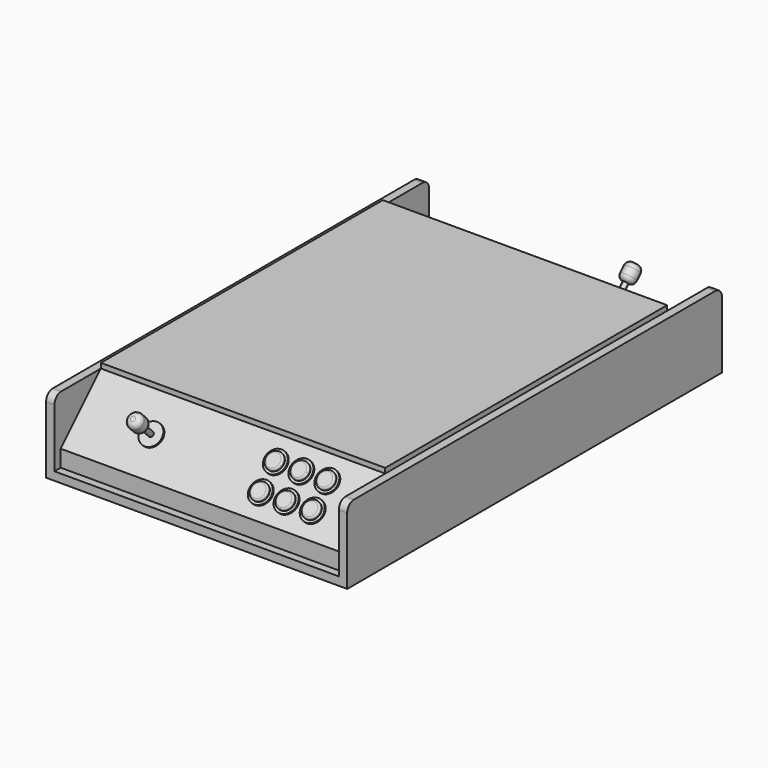
from build123d import *

# Parameters (mm, degrees)
F0_W      = 457.2
F0_H      = 711.2
F1_DEPTH  = 12.7
F3_DEPTH  = 101.6
F4_W      = 431.8
F4_H      = 171.8578838676
F5_DEPTH  = 101.6
F6_SIZE   = 76.2
F7_R      = 12.7
F8_SIZE   = 76.2
F9_R      = 12.7
F11_R     = 16.51
F11_R_2   = 12.7
F12_DEPTH = 2.54
F13_DEPTH = 7.62
F14_R     = 2.54
F15_DEPTH = 2.54
F16_DEPTH = 25.4
F17_R     = 11.120165797
F18_DEPTH = 25.4
F20_R     = 16.51
F20_R_2   = 12.7
F21_DEPTH = 2.54
F22_DEPTH = 7.62
F23_R     = 2.54
F24_DEPTH = 2.54
F25_DEPTH = 25.4
F26_R     = 11.1201708
F27_DEPTH = 25.4
F10_W     = 431.8
F10_H     = 496.0420746356
F29_DEPTH = 101.6
F30_W     = 412.6160778105
F30_H     = 477.2938070819
F31_DEPTH = 101.6
F32_SIZE2 = 61.2531853898
F32_SIZE  = 228.6
F33_W     = 431.8
F33_H     = 535.0315354705
F34_DEPTH = 7.62


# Not quite as in the source:
# - a fillet or chamfer that OpenCascade refuses, or shapes differently, is made with other operations: its cross-section is extruded or revolved along the edge and cut away or added


with BuildPart() as f1:
    # F0 (on Top) → F1 (new body)
    with BuildSketch(Plane.XY):
        with Locations((-174.0402644813, 227.3841096222)):
            Rectangle(F0_W, F0_H)
    extrude(amount=F1_DEPTH)

    # F2 (on face) → F3 (join)
    with BuildSketch(Plane.XY.offset(12.7)):
        Polygon((54.5597355187, 570.2841096222), (54.5597355187, 582.9841096222), (41.8597355187, 582.9841096222), (41.8597355187, -128.2158903778), (54.5597355187, -128.2158903778), (54.5597355187, -115.5158903778), align=None)
        Polygon((-389.9402644813, 582.9841096222), (-402.6402644813, 582.9841096222), (-402.6402644813, 570.2841096222), (-402.6402644813, -115.5158903778), (-402.6402644813, -128.2158903778), (-389.9402644813, -128.2158903778), align=None)
    extrude(amount=F3_DEPTH)

    # F4 (on face) → F5 (join)
    with BuildSketch(Plane.XY.offset(12.7)):
        with Locations((-174.0402644813, 485.1709354237)):
            Rectangle(F4_W, F4_H)
        Polygon((41.8597355187, 227.3841096222), (41.8597355187, 399.2419934899), (-389.9402644813, 399.2419934899), (-389.9402644813, 227.3841096222), (-389.9402644813, 55.5262257546), (41.8597355187, 55.5262257546), align=None)
        with Locations((-174.0402644813, -30.4027161792)):
            Rectangle(F4_W, F4_H)
    extrude(amount=F5_DEPTH)

    # F6
    f6_edges = [f1.edges().sort_by_distance(p)[0] for p in [
        (-174.040264, 571.099877, 114.3),
    ]]
    chamfer(f6_edges, length=F6_SIZE)

    # F7
    f7_edges = [f1.edges().sort_by_distance(p)[0] for p in [
        (-396.290264, 582.98411, 114.3),
        (48.209736, 582.98411, 114.3),
    ]]
    fillet(f7_edges, radius=F7_R)

    # F8
    f8_edges = [f1.edges().sort_by_distance(p)[0] for p in [
        (-174.040264, -116.331658, 114.3),
    ]]
    chamfer(f8_edges, length=F8_SIZE)

    # F9
    f9_edges = [f1.edges().sort_by_distance(p)[0] for p in [
        (-396.290264, -128.21589, 114.3),
        (48.209736, -128.21589, 114.3),
    ]]
    fillet(f9_edges, radius=F9_R)

    # F11 (on face) → F12 (join)
    with BuildSketch(Plane(origin=(0, 304.5999386787, 304.5999386787), x_dir=(-1, 0, 0), z_dir=(0, 0.7071067812, 0.7071067812))):
        with Locations((245.9873259068, -301.1169731617)):
            Circle(F11_R)
        with Locations((245.9873259068, -301.1169731617)):
            Circle(F11_R_2, mode=Mode.SUBTRACT)
        with BuildLine():
            ThreePointArc((298.5002644813, -301.1169731617), (293.6645974387, -289.4426402043), (281.9902644813, -284.6069731617))
            Line((281.9902644813, -284.6069731617), (281.9902644813, -288.4169731617))
            ThreePointArc((281.9902644813, -288.4169731617), (290.9705206024, -292.1367170406), (294.6902644813, -301.1169731617))
            ThreePointArc((294.6902644813, -301.1169731617), (290.9705206024, -310.0972292828), (281.9902644813, -313.8169731617))
            Line((281.9902644813, -313.8169731617), (281.9902644813, -317.6269731617))
            ThreePointArc((281.9902644813, -317.6269731617), (293.6645974387, -312.7913061191), (298.5002644813, -301.1169731617))
        make_face()
        with BuildLine():
            Line((281.9902644813, -288.4169731617), (281.9902644813, -284.6069731617))
            ThreePointArc((281.9902644813, -284.6069731617), (265.4802644813, -301.1169731617), (281.9902644813, -317.6269731617))
            Line((281.9902644813, -317.6269731617), (281.9902644813, -313.8169731617))
            ThreePointArc((281.9902644813, -313.8169731617), (269.2902644813, -301.1169731617), (281.9902644813, -288.4169731617))
        make_face()
        with Locations((319.3984925747, -301.1169731617)):
            Circle(F11_R)
        with Locations((319.3984925747, -301.1169731617)):
            Circle(F11_R_2, mode=Mode.SUBTRACT)
        with Locations((319.3984925747, -340.282201767)):
            Circle(F11_R)
        with Locations((319.3984925747, -340.282201767)):
            Circle(F11_R_2, mode=Mode.SUBTRACT)
        with BuildLine():
            ThreePointArc((298.5002644813, -340.282201767), (293.6645974387, -328.6078688096), (281.9902644813, -323.772201767))
            Line((281.9902644813, -323.772201767), (281.9902644813, -327.582201767))
            ThreePointArc((281.9902644813, -327.582201767), (290.9705206024, -331.3019456459), (294.6902644813, -340.282201767))
            ThreePointArc((294.6902644813, -340.282201767), (290.9705206024, -349.262457888), (281.9902644813, -352.982201767))
            Line((281.9902644813, -352.982201767), (281.9902644813, -356.792201767))
            ThreePointArc((281.9902644813, -356.792201767), (293.6645974387, -351.9565347244), (298.5002644813, -340.282201767))
        make_face()
        with BuildLine():
            Line((281.9902644813, -327.582201767), (281.9902644813, -323.772201767))
            ThreePointArc((281.9902644813, -323.772201767), (265.4802644813, -340.282201767), (281.9902644813, -356.792201767))
            Line((281.9902644813, -356.792201767), (281.9902644813, -352.982201767))
            ThreePointArc((281.9902644813, -352.982201767), (269.2902644813, -340.282201767), (281.9902644813, -327.582201767))
        make_face()
        with Locations((245.9873259068, -340.282201767)):
            Circle(F11_R)
        with Locations((245.9873259068, -340.282201767)):
            Circle(F11_R_2, mode=Mode.SUBTRACT)
    extrude(amount=F12_DEPTH)

    # F11 (on face) → F13 (join)
    with BuildSketch(Plane(origin=(0, 304.5999386787, 304.5999386787), x_dir=(-1, 0, 0), z_dir=(0, 0.7071067812, 0.7071067812))):
        with Locations((245.9873259068, -301.1169731617)):
            Circle(F11_R_2)
        with BuildLine():
            ThreePointArc((294.6902644813, -301.1169731617), (290.9705206024, -292.1367170406), (281.9902644813, -288.4169731617))
            Line((281.9902644813, -288.4169731617), (281.9902644813, -313.8169731617))
            ThreePointArc((281.9902644813, -313.8169731617), (290.9705206024, -310.0972292828), (294.6902644813, -301.1169731617))
        make_face()
        with BuildLine():
            Line((281.9902644813, -313.8169731617), (281.9902644813, -288.4169731617))
            ThreePointArc((281.9902644813, -288.4169731617), (269.2902644813, -301.1169731617), (281.9902644813, -313.8169731617))
        make_face()
        with Locations((319.3984925747, -301.1169731617)):
            Circle(F11_R_2)
        with Locations((319.3984925747, -340.282201767)):
            Circle(F11_R_2)
        with BuildLine():
            ThreePointArc((294.6902644813, -340.282201767), (290.9705206024, -331.3019456459), (281.9902644813, -327.582201767))
            Line((281.9902644813, -327.582201767), (281.9902644813, -352.982201767))
            ThreePointArc((281.9902644813, -352.982201767), (290.9705206024, -349.262457888), (294.6902644813, -340.282201767))
        make_face()
        with BuildLine():
            Line((281.9902644813, -352.982201767), (281.9902644813, -327.582201767))
            ThreePointArc((281.9902644813, -327.582201767), (269.2902644813, -340.282201767), (281.9902644813, -352.982201767))
        make_face()
        with Locations((245.9873259068, -340.282201767)):
            Circle(F11_R_2)
    extrude(amount=F13_DEPTH)

    # F14
    f14_edges = [f1.edges().sort_by_distance(p)[0] for p in [
        (-281.990264, 559.584201, 60.391984),
        (-306.698493, 550.603945, 69.37224),
        (-306.698493, 522.909946, 97.066239),
        (-281.990264, 531.890202, 88.085983),
        (-233.287326, 522.909946, 97.066239),
        (-233.287326, 550.603945, 69.37224),
    ]]
    fillet(f14_edges, radius=F14_R)

    # F11 (on face) → F15 (join)
    with BuildSketch(Plane(origin=(0, 304.5999386787, 304.5999386787), x_dir=(-1, 0, 0), z_dir=(0, 0.7071067812, 0.7071067812))):
        with BuildLine():
            Line((69.9002644813, -323.0062909247), (82.6002644813, -323.0062909247))
            ThreePointArc((82.6002644813, -323.0062909247), (77.7645974387, -311.3319579673), (66.0902644813, -306.4962909247))
            Line((66.0902644813, -306.4962909247), (66.0902644813, -319.1962909247))
            ThreePointArc((66.0902644813, -319.1962909247), (68.7843413176, -320.3122140883), (69.9002644813, -323.0062909247))
        make_face()
        with BuildLine():
            Line((66.0902644813, -319.1962909247), (66.0902644813, -306.4962909247))
            ThreePointArc((66.0902644813, -306.4962909247), (54.4159315239, -311.3319579673), (49.5802644813, -323.0062909247))
            Line((49.5802644813, -323.0062909247), (62.2802644813, -323.0062909247))
            ThreePointArc((62.2802644813, -323.0062909247), (63.396187645, -320.3122140883), (66.0902644813, -319.1962909247))
        make_face()
        with BuildLine():
            ThreePointArc((49.5802644813, -323.0062909247), (54.4159315239, -334.680623882), (66.0902644813, -339.5162909247))
            Line((66.0902644813, -339.5162909247), (66.0902644813, -326.8162909247))
            ThreePointArc((66.0902644813, -326.8162909247), (63.396187645, -325.700367761), (62.2802644813, -323.0062909247))
            Line((62.2802644813, -323.0062909247), (49.5802644813, -323.0062909247))
        make_face()
        with BuildLine():
            ThreePointArc((66.0902644813, -339.5162909247), (77.7645974387, -334.680623882), (82.6002644813, -323.0062909247))
            Line((82.6002644813, -323.0062909247), (69.9002644813, -323.0062909247))
            ThreePointArc((69.9002644813, -323.0062909247), (68.7843413176, -325.700367761), (66.0902644813, -326.8162909247))
            Line((66.0902644813, -326.8162909247), (66.0902644813, -339.5162909247))
        make_face()
    extrude(amount=F15_DEPTH)

    # F11 (on face) → F16 (join)
    with BuildSketch(Plane(origin=(0, 304.5999386787, 304.5999386787), x_dir=(-1, 0, 0), z_dir=(0, 0.7071067812, 0.7071067812))):
        with BuildLine():
            ThreePointArc((66.0902644813, -326.8162909247), (68.7843413176, -325.700367761), (69.9002644813, -323.0062909247))
            Line((69.9002644813, -323.0062909247), (66.0902644813, -323.0062909247))
            Line((66.0902644813, -323.0062909247), (66.0902644813, -326.8162909247))
        make_face()
        with BuildLine():
            Line((66.0902644813, -323.0062909247), (69.9002644813, -323.0062909247))
            ThreePointArc((69.9002644813, -323.0062909247), (68.7843413176, -320.3122140883), (66.0902644813, -319.1962909247))
            Line((66.0902644813, -319.1962909247), (66.0902644813, -323.0062909247))
        make_face()
        with BuildLine():
            Line((66.0902644813, -323.0062909247), (66.0902644813, -319.1962909247))
            ThreePointArc((66.0902644813, -319.1962909247), (63.396187645, -320.3122140883), (62.2802644813, -323.0062909247))
            Line((62.2802644813, -323.0062909247), (66.0902644813, -323.0062909247))
        make_face()
        with BuildLine():
            Line((66.0902644813, -326.8162909247), (66.0902644813, -323.0062909247))
            Line((66.0902644813, -323.0062909247), (62.2802644813, -323.0062909247))
            ThreePointArc((62.2802644813, -323.0062909247), (63.396187645, -325.700367761), (66.0902644813, -326.8162909247))
        make_face()
    extrude(amount=F16_DEPTH)

    # F17 (on face) → F18 (join)
    with BuildSketch(Plane(origin=(0, 322.5604509209, 322.5604509209), x_dir=(-1, 0, 0), z_dir=(0, 0.7071067812, 0.7071067812))):
        with Locations((66.0902644813, -323.0062909247)):
            Circle(F17_R)
    extrude(amount=F18_DEPTH)

    # F19: fillet of radius 7.62 on 2 edges, made by hand

    # F19_s1 → F19_t2 (revolve, cut)
    with BuildSketch(Plane(origin=(0, 228.3999386787, -228.3999386787), x_dir=(1, 0, 0), z_dir=(0, 0.7071067812, -0.7071067812))):
        with BuildLine():
            ThreePointArc((-77.2104302783, -473.9493643775), (-74.9785839509, -479.3375180501), (-69.5904302783, -481.5693643775))
            Line((-69.5904302783, -481.5693643775), (-77.2104302783, -481.5693643775))
            Line((-77.2104302783, -481.5693643775), (-77.2104302783, -473.9493643775))
        make_face()
    revolve(axis=Axis((-66.0902644813, 568.9209018418, 112.1210244843), (0, 0.7071067812, 0.7071067812)), mode=Mode.SUBTRACT)

    # F19_s3 → F19_t4 (revolve, cut)
    with BuildSketch(Plane(origin=(0, 228.3999386787, -228.3999386787), x_dir=(1, 0, 0), z_dir=(0, 0.7071067812, -0.7071067812))):
        with BuildLine():
            ThreePointArc((-77.2104302783, -463.7830627407), (-75.0870354409, -458.5055887535), (-69.9002644813, -456.1693643775))
            Line((-69.9002644813, -456.1693643775), (-77.2104302783, -456.1693643775))
            Line((-77.2104302783, -456.1693643775), (-77.2104302783, -463.7830627407))
        make_face()
    revolve(axis=Axis((-66.0902644813, 550.9603895996, 94.1605122421), (0, 0.7071067812, 0.7071067812)), mode=Mode.SUBTRACT)

    # F20 (on face) → F21 (join)
    with BuildSketch(Plane(origin=(0, -77.2158290565, 77.2158290565), x_dir=(1, 0, 0), z_dir=(0, -0.7071067812, 0.7071067812))):
        with Locations((-104.9405261874, 19.4476731122)):
            Circle(F20_R)
        with Locations((-104.9405261874, 19.4476731122)):
            Circle(F20_R_2, mode=Mode.SUBTRACT)
        with BuildLine():
            Line((-66.0902644813, 32.1476731122), (-66.0902644813, 35.9576731122))
            ThreePointArc((-66.0902644813, 35.9576731122), (-82.6002644813, 19.4476731122), (-66.0902644813, 2.9376731122))
            Line((-66.0902644813, 2.9376731122), (-66.0902644813, 6.7476731122))
            ThreePointArc((-66.0902644813, 6.7476731122), (-78.7902644813, 19.4476731122), (-66.0902644813, 32.1476731122))
        make_face()
        with BuildLine():
            ThreePointArc((-49.5802644813, 19.4476731122), (-54.4159315239, 31.1220060695), (-66.0902644813, 35.9576731122))
            Line((-66.0902644813, 35.9576731122), (-66.0902644813, 32.1476731122))
            ThreePointArc((-66.0902644813, 32.1476731122), (-57.1100083602, 28.4279292332), (-53.3902644813, 19.4476731122))
            ThreePointArc((-53.3902644813, 19.4476731122), (-57.1100083602, 10.4674169911), (-66.0902644813, 6.7476731122))
            Line((-66.0902644813, 6.7476731122), (-66.0902644813, 2.9376731122))
            ThreePointArc((-66.0902644813, 2.9376731122), (-54.4159315239, 7.7733401548), (-49.5802644813, 19.4476731122))
        make_face()
        with Locations((-26.6769528389, 19.4476731122)):
            Circle(F20_R)
        with Locations((-26.6769528389, 19.4476731122)):
            Circle(F20_R_2, mode=Mode.SUBTRACT)
        with Locations((-26.4120857918, -20.3579973339)):
            Circle(F20_R)
        with Locations((-26.4120857918, -20.3579973339)):
            Circle(F20_R_2, mode=Mode.SUBTRACT)
        with BuildLine():
            ThreePointArc((-49.3119074805, -20.8824866926), (-54.2428417601, -9.1136576497), (-66.0902644813, -4.3746678022))
            Line((-66.0902644813, -4.3746678022), (-66.0902644813, -8.1853222643))
            ThreePointArc((-66.0902644813, -8.1853222643), (-56.9370364603, -11.8078480246), (-53.1219074805, -20.8824866926))
            ThreePointArc((-53.1219074805, -20.8824866926), (-56.9370364603, -29.9571253607), (-66.0902644813, -33.579651121))
            Line((-66.0902644813, -33.579651121), (-66.0902644813, -37.3903055831))
            ThreePointArc((-66.0902644813, -37.3903055831), (-54.2428417601, -32.6513157356), (-49.3119074805, -20.8824866926))
        make_face()
        with BuildLine():
            Line((-66.0902644813, -8.1853222643), (-66.0902644813, -4.3746678022))
            ThreePointArc((-66.0902644813, -4.3746678022), (-82.3319074805, -20.8824866926), (-66.0902644813, -37.3903055831))
            Line((-66.0902644813, -37.3903055831), (-66.0902644813, -33.579651121))
            ThreePointArc((-66.0902644813, -33.579651121), (-78.5219074805, -20.8824866926), (-66.0902644813, -8.1853222643))
        make_face()
        with Locations((-104.6687290896, -21.3994833113)):
            Circle(F20_R)
        with Locations((-104.6687290896, -21.3994833113)):
            Circle(F20_R_2, mode=Mode.SUBTRACT)
    extrude(amount=F21_DEPTH)

    # F20 (on face) → F22 (join)
    with BuildSketch(Plane(origin=(0, -77.2158290565, 77.2158290565), x_dir=(1, 0, 0), z_dir=(0, -0.7071067812, 0.7071067812))):
        with Locations((-104.9405261874, 19.4476731122)):
            Circle(F20_R_2)
        with BuildLine():
            Line((-66.0902644813, 6.7476731122), (-66.0902644813, 32.1476731122))
            ThreePointArc((-66.0902644813, 32.1476731122), (-78.7902644813, 19.4476731122), (-66.0902644813, 6.7476731122))
        make_face()
        with BuildLine():
            ThreePointArc((-53.3902644813, 19.4476731122), (-57.1100083602, 28.4279292332), (-66.0902644813, 32.1476731122))
            Line((-66.0902644813, 32.1476731122), (-66.0902644813, 6.7476731122))
            ThreePointArc((-66.0902644813, 6.7476731122), (-57.1100083602, 10.4674169911), (-53.3902644813, 19.4476731122))
        make_face()
        with Locations((-26.6769528389, 19.4476731122)):
            Circle(F20_R_2)
        with Locations((-26.4120857918, -20.3579973339)):
            Circle(F20_R_2)
        with BuildLine():
            ThreePointArc((-53.1219074805, -20.8824866926), (-56.9370364603, -11.8078480246), (-66.0902644813, -8.1853222643))
            Line((-66.0902644813, -8.1853222643), (-66.0902644813, -33.579651121))
            ThreePointArc((-66.0902644813, -33.579651121), (-56.9370364603, -29.9571253607), (-53.1219074805, -20.8824866926))
        make_face()
        with BuildLine():
            Line((-66.0902644813, -33.579651121), (-66.0902644813, -8.1853222643))
            ThreePointArc((-66.0902644813, -8.1853222643), (-78.5219074805, -20.8824866926), (-66.0902644813, -33.579651121))
        make_face()
        with Locations((-104.6687290896, -21.3994833113)):
            Circle(F20_R_2)
    extrude(amount=F22_DEPTH)

    # F23
    f23_edges = [f1.edges().sort_by_distance(p)[0] for p in [
        (-117.640526, -68.852401, 96.355564),
        (-66.090264, -59.872145, 105.33582),
        (-39.376953, -68.852401, 96.355564),
        (-65.55355, -106.348382, 58.859584),
        (-39.112086, -96.999261, 68.208705),
        (-117.368729, -97.735702, 67.472263),
    ]]
    fillet(f23_edges, radius=F23_R)

    # F20 (on face) → F24 (join)
    with BuildSketch(Plane(origin=(0, -77.2158290565, 77.2158290565), x_dir=(1, 0, 0), z_dir=(0, -0.7071067812, 0.7071067812))):
        with BuildLine():
            Line((-278.1802644813, -1.4365992288), (-265.4802644813, -1.4365992288))
            ThreePointArc((-265.4802644813, -1.4365992288), (-270.3159315239, 10.2377337286), (-281.9902644813, 15.0734007712))
            Line((-281.9902644813, 15.0734007712), (-281.9902644813, 2.3734007712))
            ThreePointArc((-281.9902644813, 2.3734007712), (-279.296187645, 1.2574776076), (-278.1802644813, -1.4365992288))
        make_face()
        with BuildLine():
            ThreePointArc((-281.9902644813, -17.9465992288), (-270.3159315239, -13.1109321861), (-265.4802644813, -1.4365992288))
            Line((-265.4802644813, -1.4365992288), (-278.1802644813, -1.4365992288))
            ThreePointArc((-278.1802644813, -1.4365992288), (-279.296187645, -4.1306760651), (-281.9902644813, -5.2465992288))
            Line((-281.9902644813, -5.2465992288), (-281.9902644813, -17.9465992288))
        make_face()
        with BuildLine():
            Line((-281.9902644813, 2.3734007712), (-281.9902644813, 15.0734007712))
            ThreePointArc((-281.9902644813, 15.0734007712), (-298.5002644813, -1.4365992288), (-281.9902644813, -17.9465992288))
            Line((-281.9902644813, -17.9465992288), (-281.9902644813, -5.2465992288))
            ThreePointArc((-281.9902644813, -5.2465992288), (-285.8002644813, -1.4365992288), (-281.9902644813, 2.3734007712))
        make_face()
    extrude(amount=F24_DEPTH)

    # F25 (add): a face of the model
    f25_faces = [f1.faces().sort_by_distance(p)[0] for p in [
        (-281.9902644813, -78.231658113, 76.2),
    ]]
    extrude(f25_faces, amount=F25_DEPTH)

    # F26 (on face) → F27 (join)
    with BuildSketch(Plane(origin=(0, -95.1763412986, 95.1763412986), x_dir=(1, 0, 0), z_dir=(0, -0.7071067812, 0.7071067812))):
        with Locations((-281.9902644813, -1.4365992288)):
            Circle(F26_R)
    extrude(amount=F27_DEPTH)

    # F28: fillet of radius 7.62 on 2 edges, made by hand

    # F28_s1 → F28_t2 (revolve, cut)
    with BuildSketch(Plane(origin=(0, -1.0158290565, -1.0158290565), x_dir=(1, 0, 0), z_dir=(0, -0.7071067812, -0.7071067812))):
        with BuildLine():
            ThreePointArc((-270.8700936813, 152.3796726816), (-273.1019400087, 157.7678263542), (-278.4900936813, 159.9996726816))
            Line((-278.4900936813, 159.9996726816), (-270.8700936813, 159.9996726816))
            Line((-270.8700936813, 159.9996726816), (-270.8700936813, 152.3796726816))
        make_face()
    revolve(axis=Axis((-281.9902644813, -114.1526825973, 112.1210244843), (0, -0.7071067812, 0.7071067812)), mode=Mode.SUBTRACT)

    # F28_s3 → F28_t4 (revolve, cut)
    with BuildSketch(Plane(origin=(0, -1.0158290565, -1.0158290565), x_dir=(1, 0, 0), z_dir=(0, -0.7071067812, -0.7071067812))):
        with BuildLine():
            ThreePointArc((-270.8700936813, 142.2133712484), (-272.9934902526, 136.9358954552), (-278.1802644813, 134.5996726816))
            Line((-278.1802644813, 134.5996726816), (-270.8700936813, 134.5996726816))
            Line((-270.8700936813, 134.5996726816), (-270.8700936813, 142.2133712484))
        make_face()
    revolve(axis=Axis((-281.9902644813, -96.1921703551, 94.1605122421), (0, -0.7071067812, 0.7071067812)), mode=Mode.SUBTRACT)

    # F10 (on face) → F29 (cut)
    with BuildSketch(Plane.XY.offset(114.3)):
        with Locations((-174.0402644813, 227.3237099871)):
            Rectangle(F10_W, F10_H)
    extrude(amount=-F29_DEPTH, mode=Mode.SUBTRACT)

    # F30 (on face) → F31 (join)
    with BuildSketch(Plane.XY.offset(12.7)):
        with Locations((-174.9151330441, 226.3893694617)):
            Rectangle(F30_W, F30_H)
    extrude(amount=F31_DEPTH)

    # F32
    f32_edges = [f1.edges().sort_by_distance(p)[0] for p in [
        (-174.915133, 465.036273, 114.3),
        (-174.915133, -12.257534, 114.3),
    ]]
    f32_side = f1.faces().sort_by_distance((-174.915133, 226.389369, 114.3))[0]
    chamfer(f32_edges, length=F32_SIZE, length2=F32_SIZE2, reference=f32_side)


with BuildPart() as f34:
    # F33 (on face) → F34 (new body)
    with BuildSketch(Plane.XY.offset(114.3)):
        with Locations((-174.0402644813, 227.3841096222)):
            Rectangle(F33_W, F33_H)
    extrude(amount=F34_DEPTH)


solid = Compound([f1.part, f34.part])
